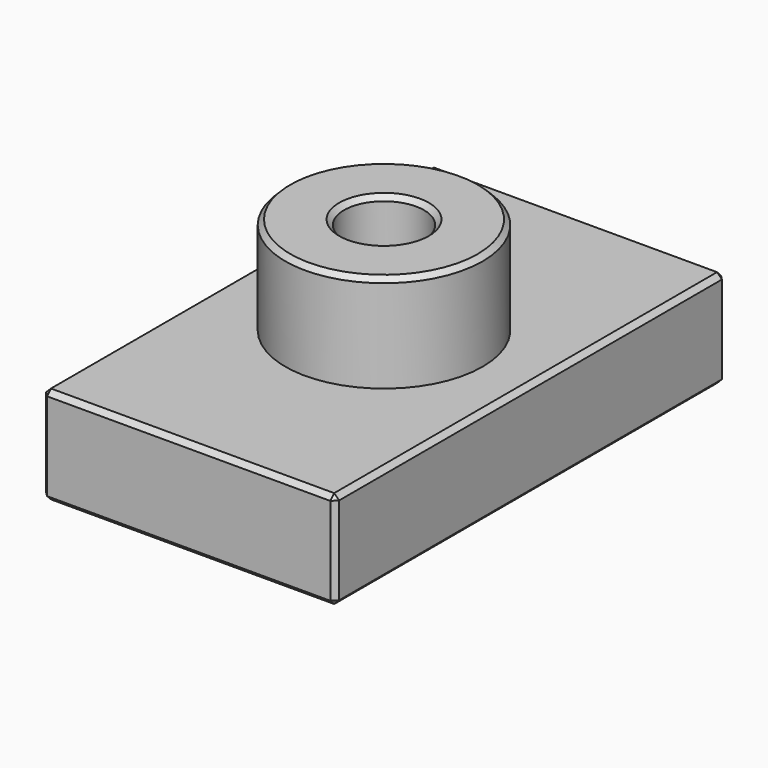
from build123d import *

# Parameters (mm, degrees)
F0_W          = 30
F0_H          = 50
F1_DEPTH      = 10
F2_R          = 10.0991386475
F3_DEPTH      = 10
F4_R          = 4.0969126616
F5_DEPTH      = 25
F5_DEPTH_BACK = 25
F6_SIZE       = 0.5
F7_SIZE       = 0.5


# Not quite as in the source:
# - a feature names something its author has since deleted; it is built from what else it names


with BuildPart() as f1:
    # F0 (on Top) → F1 (new body)
    with BuildSketch(Plane.XY):
        Rectangle(F0_W, F0_H)
    extrude(amount=-F1_DEPTH)

    # F2 (on Top) → F3 (join)
    with BuildSketch(Plane.XY):
        Circle(F2_R)
    extrude(amount=F3_DEPTH)

    # F4 (on Top) → F5 (cut, two sides)
    with BuildSketch(Plane.XY) as f5_sk:
        Circle(F4_R)
    extrude(amount=-F5_DEPTH, mode=Mode.SUBTRACT)
    extrude(f5_sk.sketch, amount=F5_DEPTH_BACK, mode=Mode.SUBTRACT)

    # F6
    f6_edges = [f1.edges().sort_by_distance(p)[0] for p in [
        (15, 0, 0),
        (0, -25, 0),
        (-15, 0, 0),
        (0, 25, 0),
        (-10.099139, 0, 10),
        (-4.096913, 0, 10),
        (15, -25, -5),
        (15, 25, -5),
        (-15, -25, -5),
        (0, -25, -10),
        (15, 0, -10),
        (-15, 25, -5),
        (-15, 0, -10),
        (0, 25, -10),
    ]]
    chamfer(f6_edges, length=F6_SIZE)

    # F7
    f7_edges = [f1.edges().sort_by_distance(p)[0] for p in [
        (-4.096913, 0, -10),
    ]]
    chamfer(f7_edges, length=F7_SIZE)


solid = f1.part
